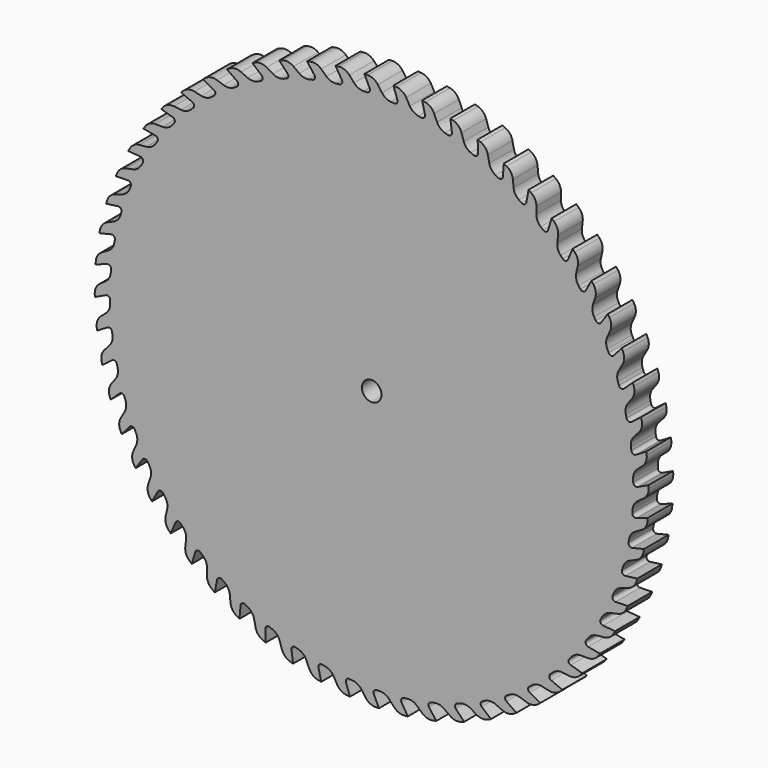
from build123d import *

# Parameters (mm, degrees)
F0_R            = 45
F1_DEPTH        = 5
F4_DEPTH        = 25
F4_COPIES_COUNT = 60
F5_R            = 2
F6_R            = 0.5
F7_R            = 1.5875
F8_DEPTH        = 25


# Not quite as in the source:
# - a pattern or mirror of a feature is missing from the dataset's text; its kind, count and spacing are read off the source's solid


with BuildPart() as f1:
    # F0 (on Front) → F1 (new body)
    with BuildSketch(Plane.XZ):
        Circle(F0_R)
    extrude(amount=F1_DEPTH)

    # F2 (on face) → F4 (cut)
    with BuildSketch(Plane.XZ.offset(5)):
        with BuildLine():
            Line((-4.3130588634, 44.7928289265), (-2.2242781403, 42.4417552271))
            ThreePointArc((-2.2242781403, 42.4417552271), (-1.1125203031, 42.4854363115), (0, 42.5))
            Line((0, 42.5), (-1.1779626739, 44.9845796239))
            ThreePointArc((-1.1779626739, 44.9845796239), (-2.7471842791, 44.916065929), (-4.3130588634, 44.7928289265))
        make_face()
    f4 = extrude(amount=-F4_DEPTH, mode=Mode.SUBTRACT)

    # F4_copies: F4 ×60 about axis
    f4_copies_axis = Axis((0, 0, 0), (0, 1, 0))
    for i in range(1, F4_COPIES_COUNT):
        add(f4.rotate(f4_copies_axis, i * 360 / F4_COPIES_COUNT), mode=Mode.SUBTRACT)

    # F5
    f5_edges = [f1.edges().sort_by_distance(p)[0] for p in [
        (-4.313059, -2.5, 44.792829),
        (-2.224278, -2.5, 42.441755),
        (0.392694, -2.5, 44.998287),
        (2.224278, -2.5, 42.441755),
        (5.094145, -2.5, 44.710734),
        (6.648465, -2.5, 41.976754),
        (9.739783, -2.5, 43.93332),
        (10.999809, -2.5, 41.051848),
        (14.27871, -2.5, 42.674564),
        (15.230638, -2.5, 39.677168),
        (18.661196, -2.5, 40.948257),
        (19.294596, -2.5, 37.867777),
        (22.839226, -2.5, 38.773312),
        (23.147159, -2.5, 35.643499),
        (26.767025, -2.5, 36.173559),
        (26.746117, -2.5, 33.028703),
        (30.401559, -2.5, 33.17748),
        (30.052038, -2.5, 30.052038),
        (33.703007, -2.5, 29.817902),
        (33.028703, -2.5, 26.746117),
        (36.635198, -2.5, 26.131633),
        (35.643499, -2.5, 23.147159),
        (39.166006, -2.5, 22.15906),
        (37.867777, -2.5, 19.294596),
        (41.267703, -2.5, 17.943708),
        (39.677168, -2.5, 15.230638),
        (42.917263, -2.5, 13.531761),
        (41.051848, -2.5, 10.999809),
        (44.096612, -2.5, 8.971557),
        (41.976754, -2.5, 6.648465),
        (44.792829, -2.5, 4.313059),
        (42.441755, -2.5, 2.224278),
        (44.998287, -2.5, -0.392694),
        (42.441755, -2.5, -2.224278),
        (44.710734, -2.5, -5.094145),
        (41.976754, -2.5, -6.648465),
        (43.93332, -2.5, -9.739783),
        (41.051848, -2.5, -10.999809),
        (42.674564, -2.5, -14.27871),
        (39.677168, -2.5, -15.230638),
        (40.948257, -2.5, -18.661196),
        (37.867777, -2.5, -19.294596),
        (38.773312, -2.5, -22.839226),
        (35.643499, -2.5, -23.147159),
        (36.173559, -2.5, -26.767025),
        (33.028703, -2.5, -26.746117),
        (33.17748, -2.5, -30.401559),
        (30.052038, -2.5, -30.052038),
        (29.817902, -2.5, -33.703007),
        (26.746117, -2.5, -33.028703),
        (26.131633, -2.5, -36.635198),
        (23.147159, -2.5, -35.643499),
        (22.15906, -2.5, -39.166006),
        (19.294596, -2.5, -37.867777),
        (17.943708, -2.5, -41.267703),
        (15.230638, -2.5, -39.677168),
        (13.531761, -2.5, -42.917263),
        (10.999809, -2.5, -41.051848),
        (8.971557, -2.5, -44.096612),
        (6.648465, -2.5, -41.976754),
        (4.313059, -2.5, -44.792829),
        (2.224278, -2.5, -42.441755),
        (-0.392694, -2.5, -44.998287),
        (-2.224278, -2.5, -42.441755),
        (-5.094145, -2.5, -44.710734),
        (-6.648465, -2.5, -41.976754),
        (-9.739783, -2.5, -43.93332),
        (-10.999809, -2.5, -41.051848),
        (-14.27871, -2.5, -42.674564),
        (-15.230638, -2.5, -39.677168),
        (-18.661196, -2.5, -40.948257),
        (-19.294596, -2.5, -37.867777),
        (-22.839226, -2.5, -38.773312),
        (-23.147159, -2.5, -35.643499),
        (-26.767025, -2.5, -36.173559),
        (-26.746117, -2.5, -33.028703),
        (-30.401559, -2.5, -33.17748),
        (-30.052038, -2.5, -30.052038),
        (-33.703007, -2.5, -29.817902),
        (-33.028703, -2.5, -26.746117),
        (-36.635198, -2.5, -26.131633),
        (-35.643499, -2.5, -23.147159),
        (-39.166006, -2.5, -22.15906),
        (-37.867777, -2.5, -19.294596),
        (-41.267703, -2.5, -17.943708),
        (-39.677168, -2.5, -15.230638),
        (-42.917263, -2.5, -13.531761),
        (-41.051848, -2.5, -10.999809),
        (-44.096612, -2.5, -8.971557),
        (-41.976754, -2.5, -6.648465),
        (-44.792829, -2.5, -4.313059),
        (-42.441755, -2.5, -2.224278),
        (-44.998287, -2.5, 0.392694),
        (-42.441755, -2.5, 2.224278),
        (-44.710734, -2.5, 5.094145),
        (-41.976754, -2.5, 6.648465),
        (-43.93332, -2.5, 9.739783),
        (-41.051848, -2.5, 10.999809),
        (-42.674564, -2.5, 14.27871),
        (-39.677168, -2.5, 15.230638),
        (-40.948257, -2.5, 18.661196),
        (-37.867777, -2.5, 19.294596),
        (-38.773312, -2.5, 22.839226),
        (-35.643499, -2.5, 23.147159),
        (-36.173559, -2.5, 26.767025),
        (-33.028703, -2.5, 26.746117),
        (-33.17748, -2.5, 30.401559),
        (-30.052038, -2.5, 30.052038),
        (-29.817902, -2.5, 33.703007),
        (-26.746117, -2.5, 33.028703),
        (-26.131633, -2.5, 36.635198),
        (-23.147159, -2.5, 35.643499),
        (-22.15906, -2.5, 39.166006),
        (-19.294596, -2.5, 37.867777),
        (-17.943708, -2.5, 41.267703),
        (-15.230638, -2.5, 39.677168),
        (-13.531761, -2.5, 42.917263),
        (-10.999809, -2.5, 41.051848),
        (-8.971557, -2.5, 44.096612),
        (-6.648465, -2.5, 41.976754),
    ]]
    fillet(f5_edges, radius=F5_R)

    # F6
    f6_edges = [f1.edges().sort_by_distance(p)[0] for p in [
        (0, -2.5, 42.5),
        (-4.44246, -2.5, 42.267181),
        (4.44246, -2.5, 42.267181),
        (-8.836247, -2.5, 41.571273),
        (8.836247, -2.5, 41.571273),
        (-13.133222, -2.5, 40.419902),
        (13.133222, -2.5, 40.419902),
        (-17.286307, -2.5, 38.825682),
        (17.286307, -2.5, 38.825682),
        (-21.25, -2.5, 36.80608),
        (21.25, -2.5, 36.80608),
        (-24.980873, -2.5, 34.383222),
        (24.980873, -2.5, 34.383222),
        (-28.438051, -2.5, 31.583655),
        (28.438051, -2.5, 31.583655),
        (-31.583655, -2.5, 28.438051),
        (31.583655, -2.5, 28.438051),
        (-34.383222, -2.5, 24.980873),
        (34.383222, -2.5, 24.980873),
        (-36.80608, -2.5, 21.25),
        (36.80608, -2.5, 21.25),
        (-38.825682, -2.5, 17.286307),
        (38.825682, -2.5, 17.286307),
        (-40.419902, -2.5, 13.133222),
        (40.419902, -2.5, 13.133222),
        (-41.571273, -2.5, 8.836247),
        (41.571273, -2.5, 8.836247),
        (-42.267181, -2.5, 4.44246),
        (42.267181, -2.5, 4.44246),
        (-42.5, -2.5, 0),
        (42.5, -2.5, 0),
        (-42.267181, -2.5, -4.44246),
        (42.267181, -2.5, -4.44246),
        (-41.571273, -2.5, -8.836247),
        (41.571273, -2.5, -8.836247),
        (-40.419902, -2.5, -13.133222),
        (40.419902, -2.5, -13.133222),
        (-38.825682, -2.5, -17.286307),
        (38.825682, -2.5, -17.286307),
        (-36.80608, -2.5, -21.25),
        (36.80608, -2.5, -21.25),
        (-34.383222, -2.5, -24.980873),
        (34.383222, -2.5, -24.980873),
        (-31.583655, -2.5, -28.438051),
        (31.583655, -2.5, -28.438051),
        (-28.438051, -2.5, -31.583655),
        (28.438051, -2.5, -31.583655),
        (-24.980873, -2.5, -34.383222),
        (24.980873, -2.5, -34.383222),
        (-21.25, -2.5, -36.80608),
        (21.25, -2.5, -36.80608),
        (-17.286307, -2.5, -38.825682),
        (17.286307, -2.5, -38.825682),
        (-13.133222, -2.5, -40.419902),
        (13.133222, -2.5, -40.419902),
        (-8.836247, -2.5, -41.571273),
        (8.836247, -2.5, -41.571273),
        (-4.44246, -2.5, -42.267181),
        (4.44246, -2.5, -42.267181),
        (0, -2.5, -42.5),
    ]]
    fillet(f6_edges, radius=F6_R)

    # F7 (on face) → F8 (cut)
    with BuildSketch(Plane.XZ.offset(5)):
        Circle(F7_R)
    extrude(amount=-F8_DEPTH, mode=Mode.SUBTRACT)


solid = f1.part
